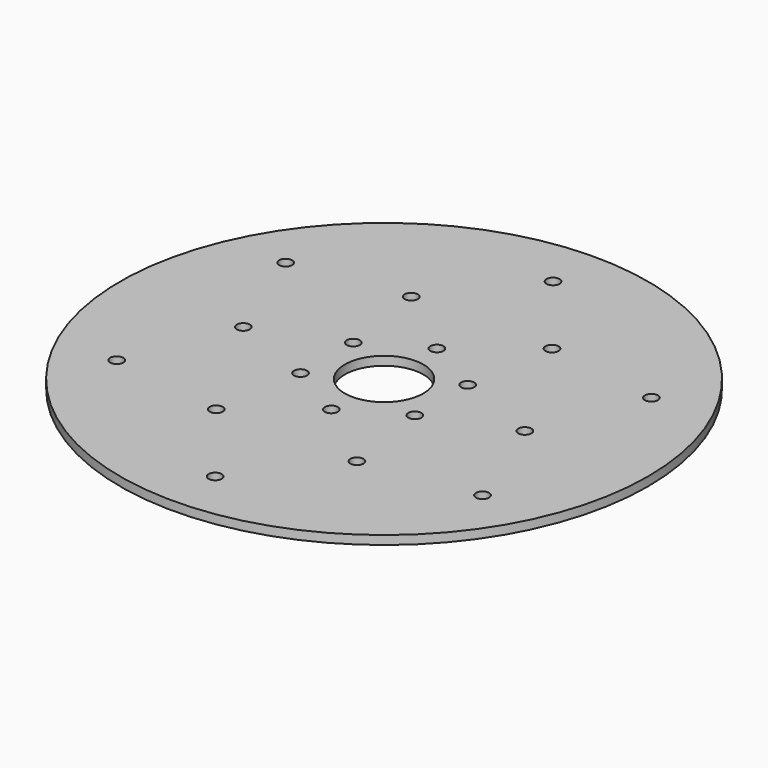
from build123d import *

# Parameters (mm, degrees)
F0_R            = 95.25
F0_R_2          = 14.1605
F1_DEPTH        = 3.175
F2_R            = 2.3622
F3_DEPTH        = 3.176
F3_COPIES_COUNT = 6


# Not quite as in the source:
# - a pattern or mirror of a feature is missing from the dataset's text; its kind, count and spacing are read off the source's solid


with BuildPart() as f1:
    # F0 (on Top) → F1 (new body)
    with BuildSketch(Plane.XY):
        Circle(F0_R)
        Circle(F0_R_2, mode=Mode.SUBTRACT)
    extrude(amount=F1_DEPTH)

    # F2 (on face) → F3 (cut, through all)
    with BuildSketch(Plane.XY.offset(3.175)):
        with Locations((0, 23.8125)):
            Circle(F2_R)
        with Locations((0, 76.2)):
            Circle(F2_R)
        with Locations((25.4, 43.9940905122)):
            Circle(F2_R)
    f3 = extrude(amount=-F3_DEPTH, mode=Mode.SUBTRACT)

    # F3_copies: F3 ×6 about axis
    f3_copies_axis = Axis((0, 0, 0), (0, 0, 1))
    for i in range(1, F3_COPIES_COUNT):
        add(f3.rotate(f3_copies_axis, i * 360 / F3_COPIES_COUNT), mode=Mode.SUBTRACT)


solid = f1.part
